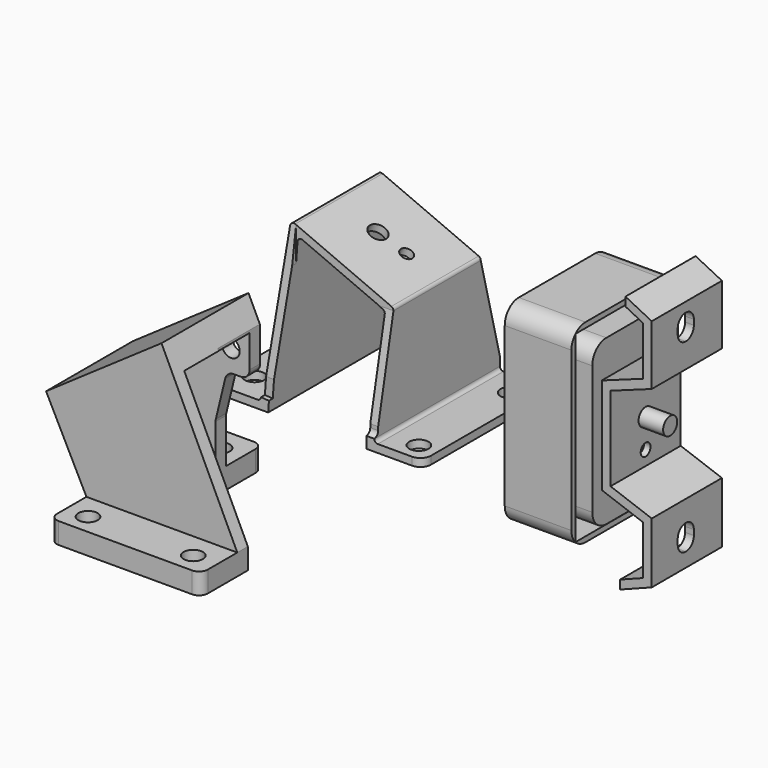
from build123d import *

# Parameters (mm, degrees)
F0_W        = 27.5
F0_H        = 4.5
F1_DEPTH    = 89.5
F2_R        = 2
F4_DEPTH    = 55.5
F5_T1_DEPTH = 4.5
F7_DEPTH    = 25
F8_R        = 5.5
F9_DEPTH    = 5
F10_R       = 5.5
F11_DEPTH   = 5
F12_R       = 5
F12_R_2     = 3.5
F13_DEPTH   = 5
F14_R       = 6
F16_DEPTH   = 61
F17_R       = 5
F18_DEPTH   = 20
F17_R_2     = 3.5
F19_DEPTH   = 2.25
F20_R       = 5
F21_DEPTH   = 26
F20_R_2     = 3.5
F22_DEPTH   = 5.5
F23_R       = 10
F25_W       = 74.5
F25_H       = 110.5
F25_R       = 5
F25_R_2     = 3.5
F26_DEPTH   = 38
F27_W       = 68.5
F27_H       = 104.5
F27_R       = 5
F27_R_2     = 3.5
F28_DEPTH   = 35
F29_R       = 10
F31_W       = 50
F31_H       = 148
F31_R       = 3.5
F31_R_2     = 5
F32_DEPTH   = 28.5
F34_DEPTH   = 50
F36_DEPTH   = 5
F38_W       = 86
F38_H       = 12
F39_DEPTH   = 62
F41_W       = 80
F41_H       = 47
F41_W_2     = 15
F42_DEPTH   = 95
F43_W       = 86
F43_H       = 12
F44_DEPTH   = 26
F45_W       = 86
F45_H       = 12
F46_DEPTH   = 26
F48_DEPTH   = 30
F50_DEPTH   = 8
F51_R       = 5
F52_R       = 5.5
F53_DEPTH   = 12
F54_R       = 5
F55_R       = 5.5
F56_DEPTH   = 25


# Not quite as in the source:
# - a fillet or chamfer that OpenCascade refuses, or shapes differently, is made with other operations: its cross-section is extruded or revolved along the edge and cut away or added


with BuildPart() as f1:
    # F0 (on Front) → F1 (new body)
    with BuildSketch(Plane.XZ):
        Polygon((-32, 0), (-27.5, 0), (-27.5, 4.5), (-27.5, 66.4633900416), (-86.0427199911, 91.6367596378), (-92.1935500832, 4.5), (-92.4888345559, 0.3168033031), (-92.5, 0), (-88, 0), (-82, 85), (-32, 63.5), align=None)
        with Locations((-13.75, 2.25)):
            Rectangle(F0_W, F0_H)
        Polygon((-120, 0), (-92.5, 0), (-92.4888345559, 0.3168033031), (-92.1935500832, 4.5), (-120, 4.5), align=None)
    extrude(amount=-F1_DEPTH)

    # F2
    f2_edges = [f1.edges().sort_by_distance(p)[0] for p in [
        (-86.04272, 44.75, 91.63676),
        (-82, 44.75, 85),
        (-32, 44.75, 63.5),
        (-27.5, 44.75, 66.46339),
        (-92.19355, 44.75, 4.5),
        (-27.5, 44.75, 4.5),
    ]]
    fillet(f2_edges, radius=F2_R)

    # F3 (on face) → F4 (cut)
    with BuildSketch(Plane.YZ.offset(-27.5)):
        Polygon((89.5, 66.9836661761), (89.5, 90.5244270628), (75.85, 90.5244270628), (75.85, 65.1463278009), (89.5, 65.1463278009), align=None)
        Polygon((89.5, 65.1463278009), (75.85, 65.1463278009), (89.5, 11.5), align=None)
        Polygon((2.75, 11.5), (13.65, 65.1463278009), (0, 65.1463278009), (0, 6.5), (2.75, 6.5), align=None)
        Polygon((13.65, 65.1463278009), (13.65, 90.5244270628), (0, 90.5244270628), (0, 66.9836661761), (0, 65.1463278009), align=None)
    extrude(amount=-F4_DEPTH, mode=Mode.SUBTRACT)

    # F5: fillet of radius 3 on 1 edges, made by hand

    # F5_s2 → F5_t1 (join)
    with BuildSketch(Plane.YZ.offset(-32)):
        with BuildLine():
            ThreePointArc((2.75, 9.4895651858), (1.9579402166, 7.4585555846), (0, 6.5))
            Line((0, 6.5), (2.75, 6.5))
            Line((2.75, 6.5), (2.75, 9.4895651858))
        make_face()
    extrude(amount=F5_T1_DEPTH)

    # F6 (on face) → F7 (cut)
    with BuildSketch(Plane(origin=(-92.0525271107, 0, 6.4978254431), x_dir=(0, -1, 0), z_dir=(-0.9975179223, 0, 0.0704130298))):
        Polygon((-89.5, 9.5350977863), (-76.1650987076, 82.5349474599), (-89.5, 82.5349474599), align=None)
        Polygon((-89.5, 84.4233556199), (-75.85, 84.4233556199), (-75.85, 87.4233556199), (-89.5, 87.4233556199), (-89.5, 84.5349474599), align=None)
        Polygon((-75.85, 84.2599064816), (-75.85, 84.4233556199), (-89.5, 84.4233556199), (-89.5, 82.5349474599), (-76.1650987076, 82.5349474599), align=None)
        Polygon((-13.65, 87.4233556199), (-13.65, 84.4233556199), (0, 84.4233556199), (0, 84.5349474599), (0, 87.4233556199), align=None)
        Polygon((-13.65, 84.4233556199), (-13.65, 84.2599064816), (-13.398382717, 82.5349474599), (0, 82.5349474599), (0, 84.4233556199), align=None)
        Polygon((0, 82.5349474599), (-13.398382717, 82.5349474599), (-2.75, 9.5350977863), (-2.75, 7.5296530276), (-2.75, -0.1389965028), (0, -0.1389965028), align=None)
    extrude(amount=-F7_DEPTH, mode=Mode.SUBTRACT)

    # F8 (on face) → F9 (cut)
    with BuildSketch(Plane.XY.offset(4.5)):
        with Locations((-10.5, 10.5)):
            Circle(F8_R)
        with Locations((-10.5, 75.5)):
            Circle(F8_R)
    extrude(amount=-F9_DEPTH, mode=Mode.SUBTRACT)

    # F10 (on face) → F11 (cut)
    with BuildSketch(Plane.XY.offset(4.5)):
        with Locations((-109, 16.5)):
            Circle(F10_R)
        with Locations((-109, 78.5)):
            Circle(F10_R)
    extrude(amount=-F11_DEPTH, mode=Mode.SUBTRACT)

    # F12 (on face) → F13 (cut)
    with BuildSketch(Plane(origin=(19.8282620625, 0, 46.1122373547), x_dir=(0.9186691876, 0, -0.3950277507), z_dir=(0.3950277507, 0, 0.9186691876))):
        with Locations((-88.3164328594, 44.85)):
            Circle(F12_R)
        with Locations((-71.8164328594, 46.35)):
            Circle(F12_R_2)
    extrude(amount=-F13_DEPTH, mode=Mode.SUBTRACT)

    # F14
    f14_edges = [f1.edges().sort_by_distance(p)[0] for p in [
        (0, 89.5, 2.25),
        (0, 0, 2.25),
        (-120, 0, 2.25),
        (-120, 89.5, 2.25),
    ]]
    fillet(f14_edges, radius=F14_R)


with BuildPart() as f16:
    # F15 (on Front) → F16 (new body)
    with BuildSketch(Plane.XZ):
        Polygon((53.25, 0), (75, 0), (96.75, 0), (96.75, 93.5), (53.25, 93.5), align=None)
    extrude(amount=-F16_DEPTH)

    # F17 (on face) → F18 (join)
    with BuildSketch(Plane.YZ.offset(96.75)):
        with Locations((30.5, 47.5)):
            Circle(F17_R)
    extrude(amount=F18_DEPTH)

    # F17 (on face) → F19 (join)
    with BuildSketch(Plane.YZ.offset(96.75)):
        with Locations((30.5, 47.5)):
            Circle(F17_R)
        with Locations((30.5, 31)):
            Circle(F17_R_2)
    extrude(amount=F19_DEPTH)

    # F20 (on face) → F21 (join)
    with BuildSketch(Plane(origin=(53.25, 0, 0), x_dir=(0, -1, 0), z_dir=(-1, 0, 0))):
        with Locations((-30.5, 36.5)):
            Circle(F20_R)
    extrude(amount=F21_DEPTH)

    # F20 (on face) → F22 (join)
    with BuildSketch(Plane(origin=(53.25, 0, 0), x_dir=(0, -1, 0), z_dir=(-1, 0, 0))):
        with Locations((-30.5, 36.5)):
            Circle(F20_R)
        with Locations((-30.5, 53)):
            Circle(F20_R_2)
    extrude(amount=F22_DEPTH)

    # F23
    f23_edges = [f16.edges().sort_by_distance(p)[0] for p in [
        (75, 0, 93.5),
        (75, 61, 93.5),
        (75, 61, 0),
        (75, 0, 0),
    ]]
    fillet(f23_edges, radius=F23_R)


with BuildPart() as f26:
    # F25 (on offset) → F26 (new body)
    with BuildSketch(Plane(origin=(52.25, 0, 0), x_dir=(0, -1, 0), z_dir=(-1, 0, 0))):
        with Locations((-30.5, 46.75)):
            Rectangle(F25_W, F25_H)
        with Locations((-30.5, 36.5)):
            Circle(F25_R, mode=Mode.SUBTRACT)
        with Locations((-30.5, 53)):
            Circle(F25_R_2, mode=Mode.SUBTRACT)
    extrude(amount=-F26_DEPTH)

    # F27 (on face) → F28 (cut)
    with BuildSketch(Plane.YZ.offset(90.25)):
        with Locations((30.5, 46.75)):
            Rectangle(F27_W, F27_H)
        with Locations((30.5, 36.5)):
            Circle(F27_R, mode=Mode.SUBTRACT)
        with Locations((30.5, 53)):
            Circle(F27_R_2, mode=Mode.SUBTRACT)
    extrude(amount=-F28_DEPTH, mode=Mode.SUBTRACT)

    # F29
    f29_edges = [f26.edges().sort_by_distance(p)[0] for p in [
        (71.25, -6.75, 102),
        (71.25, 67.75, 102),
        (71.25, 67.75, -8.5),
        (71.25, -6.75, -8.5),
    ]]
    fillet(f29_edges, radius=F29_R)


with BuildPart() as f32:
    # F31 (on offset) → F32 (new body)
    with BuildSketch(Plane.YZ.offset(97.75)):
        with Locations((30.5, 46.75)):
            Rectangle(F31_W, F31_H)
        with Locations((30.5, 31)):
            Circle(F31_R, mode=Mode.SUBTRACT)
        with Locations((30.5, 47.5)):
            Circle(F31_R_2, mode=Mode.SUBTRACT)
    extrude(amount=F32_DEPTH)

    # F33 (on face) → F34 (cut)
    with BuildSketch(Plane.XZ.offset(-5.5)):
        Polygon((111.25, 120.75), (126.25, 113.25), (126.25, 120.75), align=None)
        Polygon((97.75, 120.75), (97.75, 74.25), (121.25, 82.75), (121.25, 110.75), (111.25, 115.75), (111.25, 120.75), align=None)
        Polygon((102.75, 22.7585102126), (126.25, 14.2585102126), (126.25, 79.2414897874), (102.75, 70.7414897874), align=None)
        Polygon((97.75, -27.25), (108.25, -27.25), (108.25, -22.25), (121.25, -17.25), (121.25, 10.75), (97.75, 19.25), align=None)
        Polygon((108.25, -27.25), (126.25, -27.25), (126.25, -20.3269230769), align=None)
    extrude(amount=-F34_DEPTH, mode=Mode.SUBTRACT)

    # F35 (on face) → F36 (cut)
    with BuildSketch(Plane.YZ.offset(126.25)):
        with BuildLine():
            ThreePointArc((29.75, -12.25), (33.8158639918, -10.5658639918), (35.5, -6.5))
            Line((35.5, -6.5), (35.5, -3.5))
            ThreePointArc((35.5, -3.5), (33.8158639918, 0.5658639918), (29.75, 2.25))
            ThreePointArc((29.75, 2.25), (25.6841360082, 0.5658639918), (24, -3.5))
            Line((24, -3.5), (24, -6.5))
            ThreePointArc((24, -6.5), (25.6841360082, -10.5658639918), (29.75, -12.25))
        make_face()
        with BuildLine():
            ThreePointArc((24, 99), (25.6841360082, 94.9341360082), (29.75, 93.25))
            ThreePointArc((29.75, 93.25), (33.8158639918, 94.9341360082), (35.5, 99))
            Line((35.5, 99), (35.5, 102))
            ThreePointArc((35.5, 102), (33.8158639918, 106.0658639918), (29.75, 107.75))
            ThreePointArc((29.75, 107.75), (25.6841360082, 106.0658639918), (24, 102))
            Line((24, 102), (24, 99))
        make_face()
    extrude(amount=-F36_DEPTH, mode=Mode.SUBTRACT)


with BuildPart() as f39:
    # F38 (on offset) → F39 (new body)
    with BuildSketch(Plane.XZ.offset(70)):
        with Locations((-43, 6)):
            Rectangle(F38_W, F38_H)
        Polygon((-86, 12), (0, 12), (-43.199164139, 103), (-109, 57.5), align=None)
    extrude(amount=F39_DEPTH)

    # F41 (on offset) → F42 (cut)
    with BuildSketch(Plane(origin=(-53.0576073158, 0, 76.730437586), x_dir=(0.8225104483, 0, 0.56875), z_dir=(-0.56875, 0, 0.8225104483))):
        with Locations((-16.9505138605, -101)):
            Rectangle(F41_W, F41_H)
        with Locations((-64.4505138605, -101)):
            Rectangle(F41_W_2, F41_H)
    extrude(amount=-F42_DEPTH, mode=Mode.SUBTRACT)

    # F43 (on face) → F44 (join)
    with BuildSketch(Plane.XZ.offset(132)):
        with Locations((-43, 6)):
            Rectangle(F43_W, F43_H)
    extrude(amount=F44_DEPTH)

    # F45 (on face) → F46 (join)
    with BuildSketch(Plane(origin=(0, -70, 0), x_dir=(-1, 0, 0), z_dir=(0, 1, 0))):
        with Locations((43, 6)):
            Rectangle(F45_W, F45_H)
    extrude(amount=F46_DEPTH)

    # F47 (on face) → F48 (cut, symmetric)
    with BuildSketch(Plane(origin=(0, -70, 0), x_dir=(-1, 0, 0), z_dir=(0, 1, 0))):
        Polygon((56, 38), (49.5736579711, 64.5500405693), (36.5736579711, 64.5500405693), (36.7664510416, 89.4493467978), (0, 12), (0, 0), (56, 0), (56, 12), align=None)
    extrude(amount=F48_DEPTH, both=True, mode=Mode.SUBTRACT)

    # F49 (on face) → F50 (cut)
    with BuildSketch(Plane(origin=(0, -70, 0), x_dir=(-1, 0, 0), z_dir=(0, 1, 0))):
        with BuildLine():
            ThreePointArc((52.1981022078, 77.134801483), (51.6263496037, 79.4565734356), (50.0418522078, 81.2473537243))
            ThreePointArc((50.0418522078, 81.2473537243), (42.7698548118, 74.8130295304), (52.1981022078, 77.134801483))
        make_face()
    extrude(amount=-F50_DEPTH, mode=Mode.SUBTRACT)

    # F51
    f51_edges = [f39.edges().sort_by_distance(p)[0] for p in [
        (-36.573658, -73.75, 64.550041),
        (-49.573658, -73.75, 64.550041),
        (-56, -73.75, 38),
    ]]
    fillet(f51_edges, radius=F51_R)

    # F52 (on face) → F53 (cut)
    with BuildSketch(Plane.XY.offset(12)):
        with Locations((-73.5, -146.5)):
            Circle(F52_R)
        with Locations((-13.5, -146.5)):
            Circle(F52_R)
    extrude(amount=-F53_DEPTH, mode=Mode.SUBTRACT)

    # F54
    f54_edges = [f39.edges().sort_by_distance(p)[0] for p in [
        (-86, -158, 6),
        (0, -158, 6),
        (-86, -44, 6),
        (-56, -44, 6),
    ]]
    fillet(f54_edges, radius=F54_R)

    # F55 (on face) → F56 (cut)
    with BuildSketch(Plane.XY.offset(12)):
        with Locations((-69, -58)):
            Circle(F55_R)
    extrude(amount=-F56_DEPTH, mode=Mode.SUBTRACT)


solid = Compound([f1.part, f16.part, f26.part, f32.part, f39.part])
